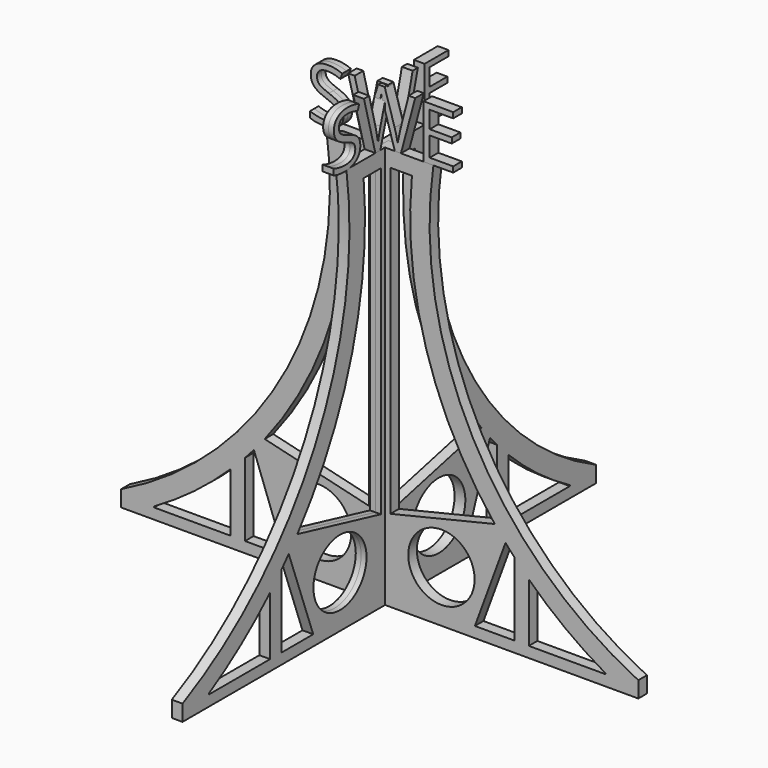
from build123d import *

# Parameters (mm, degrees)
F0_R          = 6.1806472431
F1_DEPTH      = 1
F1_DEPTH_BACK = 1
F3_COUNT      = 4
F3_ANGLE      = 270
F4_TEXT_SIZE  = 13.8888888889
F5_DEPTH      = 1
F5_DEPTH_BACK = 1
F6_TEXT_SIZE  = 13.9672550154
F7_DEPTH      = 1
F7_DEPTH_BACK = 1
F8_DEPTH      = 1
F8_DEPTH_BACK = 1


# Not quite as in the source:
# - Text() gives the source's letters only with a copy of the font that has no kerning and outlines rounded to 1/6400 em; it was checked with that copy


with BuildPart() as f1:
    # F0 (on Right) → F1 (new body, two sides)
    with BuildSketch(Plane.YZ) as f1_sk:
        with BuildLine():
            Line((0, 75), (-10, 75))
            ThreePointArc((-10, 75), (-17.3120611875, 32.7661017706), (-48.152741852, 3))
            Line((-48.152741852, 3), (-48.152741852, 0))
            Line((-48.152741852, 0), (0, 0))
            Line((0, 0), (0, 75))
        make_face()
        with BuildLine():
            Line((-27.764151271, 12.9135319579), (-27.764151271, 2))
            Line((-27.764151271, 2), (-42, 2))
            Line((-42, 2), (-42, 2.1750166227))
            ThreePointArc((-42, 2.1750166227), (-34.5511609173, 7.105586844), (-27.764151271, 12.9135319579))
        make_face(mode=Mode.SUBTRACT)
        with BuildLine():
            Line((-23.4289781128, 17.4931603787), (-17.7242412692, 2))
            Line((-17.7242412692, 2), (-25.0797602726, 2))
            Line((-25.0797602726, 2), (-25.0797602726, 15.6543289028))
            ThreePointArc((-25.0797602726, 15.6543289028), (-24.2465458174, 16.5667213281), (-23.4289781128, 17.4931603787))
        make_face(mode=Mode.SUBTRACT)
        with Locations((-11.4981485531, 9.6015622839)):
            Circle(F0_R, mode=Mode.SUBTRACT)
        with BuildLine():
            Line((-6, 72), (-2, 72))
            Line((-2, 72), (-2, 15.2730196714))
            Line((-2, 15.2730196714), (-21.4176884088, 19.9159540401))
            ThreePointArc((-21.4176884088, 19.9159540401), (-8.6548548434, 44.4619174925), (-6, 72))
        make_face(mode=Mode.SUBTRACT)
    extrude(amount=F1_DEPTH)
    extrude(f1_sk.sketch, amount=-F1_DEPTH_BACK)


with BuildPart() as f3_1:
    # F3: instance of F1
    add(f1.part.rotate(Axis((0, 0, 26.2590656057), (0, 0, -1)), 1 * F3_ANGLE / (F3_COUNT - 1)))


with BuildPart() as f3_2:
    # F3: instance of F1
    add(f1.part.rotate(Axis((0, 0, 26.2590656057), (0, 0, -1)), 2 * F3_ANGLE / (F3_COUNT - 1)))


with BuildPart() as f3_3:
    # F3: instance of F1
    add(f1.part.rotate(Axis((0, 0, 26.2590656057), (0, 0, -1)), 3 * F3_ANGLE / (F3_COUNT - 1)))


with BuildPart() as f5:
    # F4 (on Front) → F5 (new body, two sides)
    with BuildSketch(Plane.XZ) as f5_sk:
        with Locations((-13.6859809028, 75)):
            Text('SWE', F4_TEXT_SIZE, font='Open Sans', text_align=(TextAlign.LEFT, TextAlign.BOTTOM))
    extrude(amount=F5_DEPTH)
    extrude(f5_sk.sketch, amount=-F5_DEPTH_BACK)


with BuildPart() as f7:
    # F6 (on Right) → F7 (new body, two sides)
    with BuildSketch(Plane.YZ) as f7_sk:
        with Locations((-13.7632021492, 75)):
            Text('SWE', F6_TEXT_SIZE, font='Open Sans', text_align=(TextAlign.LEFT, TextAlign.BOTTOM))
    extrude(amount=F7_DEPTH)
    extrude(f7_sk.sketch, amount=-F7_DEPTH_BACK)


with BuildPart() as f8:
    # F6 (on Right) → F8 (new body, two sides)
    with BuildSketch(Plane.YZ) as f8_sk:
        with Locations((-13.7632021492, 75)):
            Text('SWE', F6_TEXT_SIZE, font='Open Sans', text_align=(TextAlign.LEFT, TextAlign.BOTTOM))
    extrude(amount=F8_DEPTH)
    extrude(f8_sk.sketch, amount=-F8_DEPTH_BACK)


solid = Compound([f1.part, f3_1.part, f3_2.part, f3_3.part, f5.part, f7.part, f8.part])
